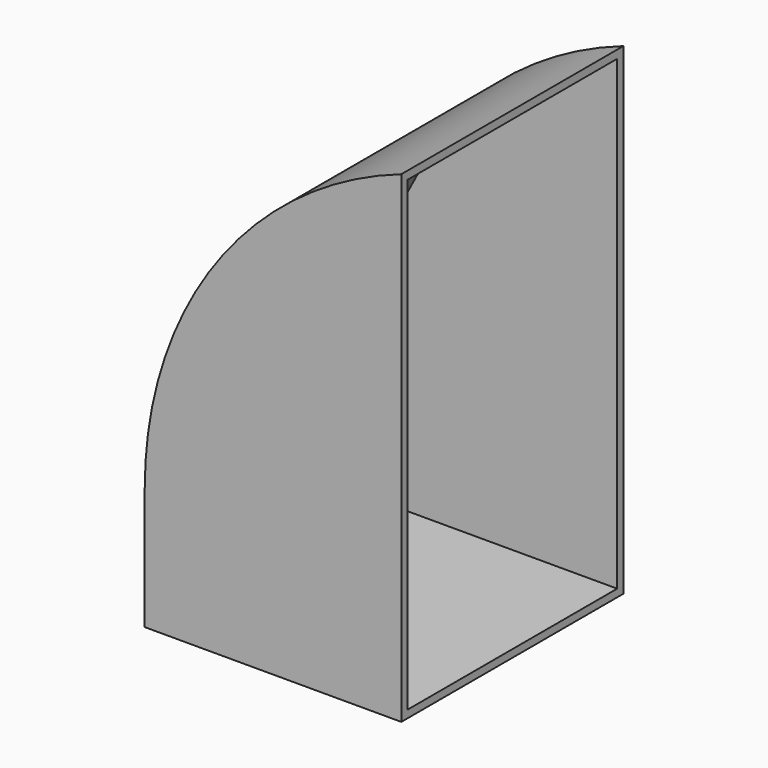
from build123d import *

# Parameters (mm, degrees)
F0_W        = 85.4306071997
F0_H        = 92.3714498058
F1_DEPTH    = 160.528
F2_T1_DEPTH = 692.3919824172
F3_T        = -2.54


# Not quite as in the source:
# - a fillet or chamfer that OpenCascade refuses, or shapes differently, is made with other operations: its cross-section is extruded or revolved along the edge and cut away or added


with BuildPart() as f1:
    # F0 (on Top) → F1 (new body)
    with BuildSketch(Plane.XY):
        with Locations((-126.2646093965, -30.766769778)):
            Rectangle(F0_W, F0_H)
    extrude(amount=F1_DEPTH)

    # F2: fillet of radius 127 on 1 edges, made by hand

    # F2_s2 → F2_t1 (cut)
    with BuildSketch(Plane.XZ.offset(-315.4292214306)):
        with BuildLine():
            ThreePointArc((-168.9799129963, 40.5238934777), (-145.4408062982, 114.1774307803), (-83.5493057966, 160.528))
            Line((-83.5493057966, 160.528), (-168.9799129963, 160.528))
            Line((-168.9799129963, 160.528), (-168.9799129963, 40.5238934777))
        make_face()
    extrude(amount=F2_T1_DEPTH, mode=Mode.SUBTRACT)

    # F3
    f3_openings = [f1.faces().sort_by_distance(p)[0] for p in [
        (-83.549306, -30.76677, 80.264),
    ]]
    offset(amount=F3_T, openings=f3_openings)


solid = f1.part
